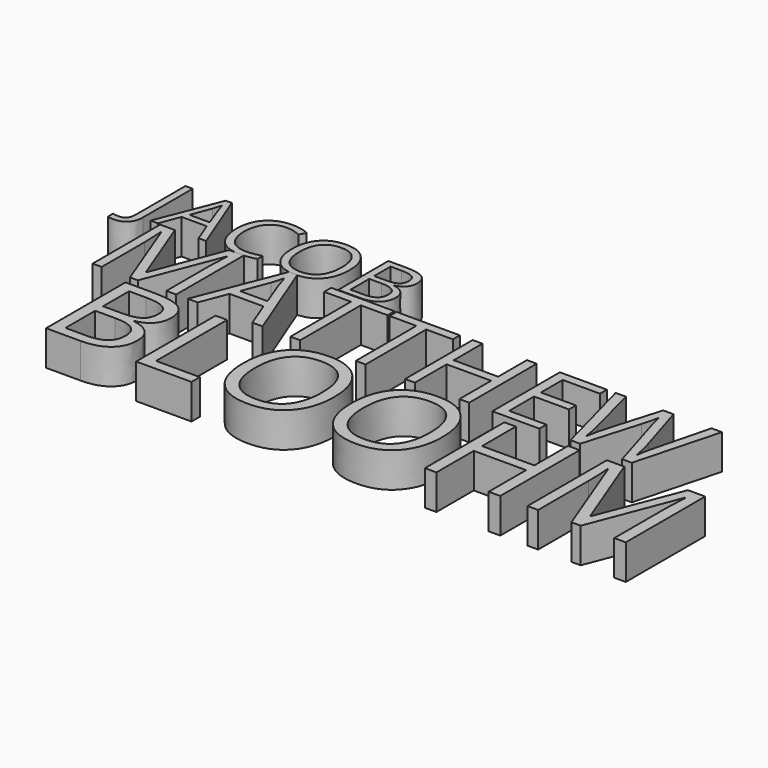
from build123d import *

# Parameters (mm, degrees)
F0_TEXT_SIZE = 63.7919745511
F1_DEPTH     = 25.4
F2_TEXT_SIZE = 86.0729461743
F3_DEPTH     = 25.4
F4_TEXT_SIZE = 101.1903397739
F5_DEPTH     = 25.4


# Not quite as in the source:
# - Text() gives the source's letters only with a copy of the font that has no kerning and outlines rounded to 1/6400 em; it was checked with that copy


with BuildPart() as f1:
    # F0 (on Top) → F1 (new body)
    with BuildSketch(Plane.XY):
        with Locations((0, 0)):
            Text('JACOB', F0_TEXT_SIZE, font='Open Sans', text_align=(TextAlign.LEFT, TextAlign.BOTTOM))
    extrude(amount=F1_DEPTH)


with BuildPart() as f3:
    # F2 (on Top) → F3 (new body)
    with BuildSketch(Plane.XY):
        with Locations((15.9248299897, -61.9725212455)):
            Text('MATTHEW', F2_TEXT_SIZE, font='Open Sans', text_align=(TextAlign.LEFT, TextAlign.BOTTOM))
    extrude(amount=F3_DEPTH)


with BuildPart() as f5:
    # F4 (on Top) → F5 (new body)
    with BuildSketch(Plane.XY):
        with Locations((43.4745810926, -140.5842006207)):
            Text('BLOOHM', F4_TEXT_SIZE, font='Open Sans', text_align=(TextAlign.LEFT, TextAlign.BOTTOM))
    extrude(amount=F5_DEPTH)


solid = Compound([f1.part, f3.part, f5.part])
